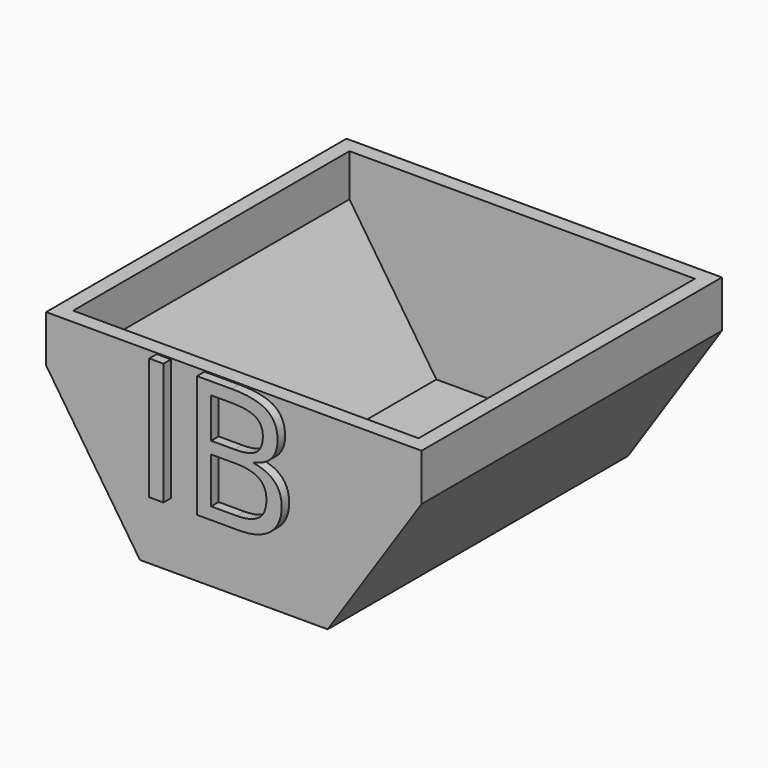
from build123d import *

# Parameters (mm, degrees)
F1_DEPTH     = 50.8
F2_T         = -2.032
F3_TEXT_SIZE = 23.1622075786
F4_DEPTH     = 1.27


# Not quite as in the source:
# - Text() gives the source's letters only with a copy of the font that has no kerning and outlines rounded to 1/6400 em; it was checked with that copy


with BuildPart() as f1:
    # F0 (on Front) → F1 (new body)
    with BuildSketch(Plane.XZ):
        Polygon((-86.5847968221, 16.6767894566), (-111.9847968221, 16.6767894566), (-111.9847968221, 10.3267894566), (-99.2847968221, -8.7232105434), (-86.5847968221, -8.7232105434), align=None)
        Polygon((-61.1847968221, 16.6767894566), (-86.5847968221, 16.6767894566), (-86.5847968221, -8.7232105434), (-73.8847968221, -8.7232105434), (-61.1847968221, 10.3267894566), align=None)
    extrude(amount=F1_DEPTH)

    # F2
    f2_openings = [f1.faces().sort_by_distance(p)[0] for p in [
        (-86.584797, -25.4, 16.676789),
    ]]
    offset(amount=F2_T, openings=f2_openings)

    # F3 (on face) → F4 (join)
    with BuildSketch(Plane.XZ.offset(50.8)):
        with Locations((-99.2847968221, 0)):
            Text('IB', F3_TEXT_SIZE, font='Open Sans', text_align=(TextAlign.LEFT, TextAlign.BOTTOM))
    extrude(amount=F4_DEPTH)


solid = f1.part
